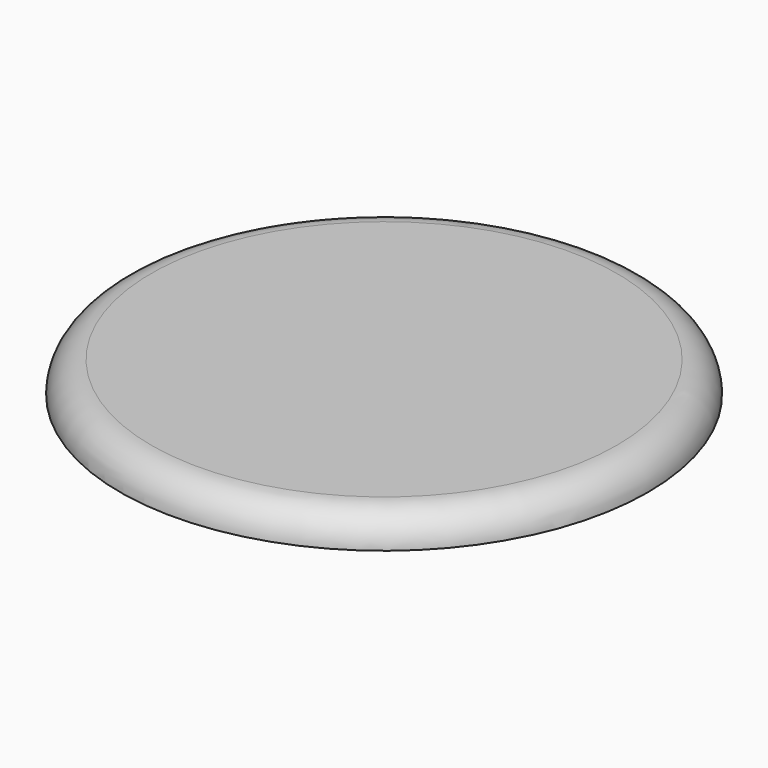
from build123d import *

# Parameters (mm, degrees)
F0_R     = 25.4
F1_DEPTH = 3
F2_R     = 2.99999


# Not quite as in the source:
# - a fillet or chamfer is up to 0.001 mm smaller than in the source, because OpenCascade refuses the exact size


with BuildPart() as f1:
    # F0 (on Top) → F1 (new body)
    with BuildSketch(Plane.XY):
        Circle(F0_R)
    extrude(amount=-F1_DEPTH)

    # F2 (radius 3 in the source; OpenCascade refuses exactly that, so slightly less here)
    f2_edges = [f1.edges().sort_by_distance(p)[0] for p in [
        (-25.4, 0, 0),
    ]]
    fillet(f2_edges, radius=F2_R)


solid = f1.part
